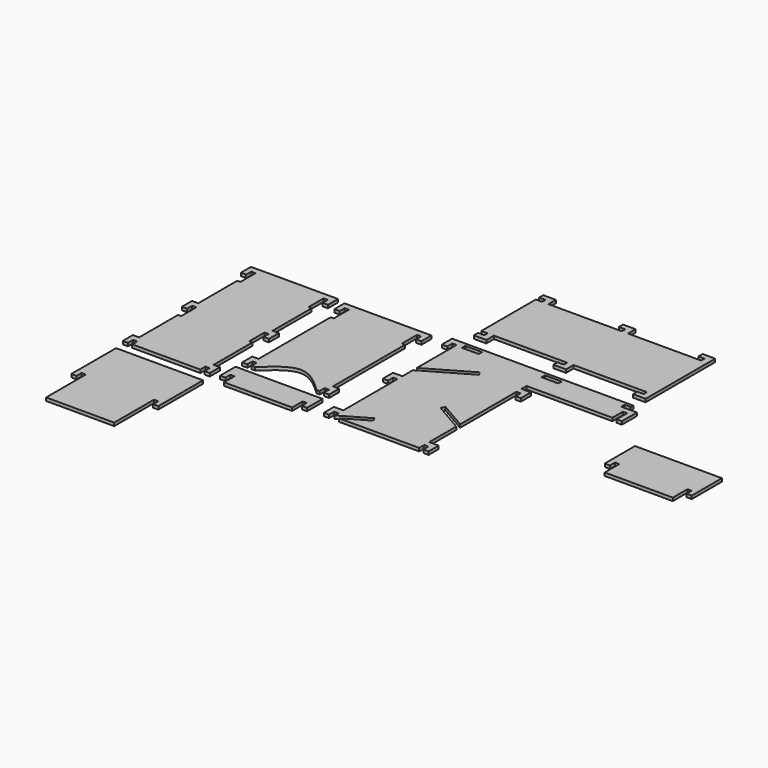
from build123d import *

# Parameters (mm, degrees)
F1_DEPTH = 3
F2_DEPTH = 3
F0_W     = 16
F0_H     = 4
F3_DEPTH = 3
F4_DEPTH = 3


with BuildPart() as f1:
    # F0 (on Top) → F1 (new body)
    with BuildSketch(Plane.XY):
        Polygon((-231.130471, -198.386263), (-231.130471, -245.736263), (-166.130471, -245.736263), (-166.130471, -198.386263), (-162.130471, -198.386263), (-162.130471, -204.386263), (-157.103619, -204.386263), (-157.103619, -151.036263), (-240.130471, -151.036263), (-240.130471, -204.386263), (-235.130471, -204.386263), (-235.130471, -198.386263), align=None)
    extrude(amount=F1_DEPTH)


with BuildPart() as f2:
    # F0 (on Top) → F2 (new body)
    with BuildSketch(Plane.XY):
        Polygon((-234.530405, -138.7419), (-169.530405, -138.7419), (-169.530405, -132.7419), (-165.530405, -132.7419), (-165.530405, -138.7419), (-160.530405, -138.7419), (-160.530405, -126.7419), (-166.530405, -126.7419), (-166.530405, -80.2419), (-169.530405, -80.2419), (-169.530405, -62.2419), (-165.530405, -62.2419), (-165.530405, -68.2419), (-160.503553, -68.2419), (-160.503553, -56.2419), (-166.530405, -56.2419), (-166.530405, -9.7419), (-169.530405, -9.7419), (-169.530405, 8.2581), (-165.530405, 8.2581), (-165.530405, 2.2581), (-160.503553, 2.2581), (-160.503553, 14.2581), (-243.530405, 14.2581), (-243.530405, 2.2581), (-238.530405, 2.2581), (-238.530405, 8.2581), (-234.530405, 8.2581), (-234.530405, -9.7419), (-237.530405, -9.7419), (-237.530405, -56.2419), (-243.530405, -56.2419), (-243.530405, -68.2419), (-238.530405, -68.2419), (-238.530405, -62.2419), (-234.530405, -62.2419), (-234.530405, -80.2419), (-237.530405, -80.2419), (-237.530405, -126.7419), (-243.530405, -126.7419), (-243.530405, -138.7419), (-238.530405, -138.7419), (-238.530405, -132.7419), (-234.530405, -132.7419), align=None)
    extrude(amount=F2_DEPTH)


with BuildPart() as f3:
    # F0 (on Top) → F3 (new body)
    with BuildSketch(Plane.XY):
        Polygon((118.848138, 17.368657), (-45.151862, 17.368657), (-54.151862, 17.368657), (-54.151862, 5.368657), (-49.151862, 5.368657), (-49.151862, 11.368657), (-45.151862, 11.368657), (-45.151862, -35.974066), (-3.989674, -12.209066), (-1.989674, -15.673167), (-45.151862, -40.592868), (-45.151862, -53.131343), (-54.151862, -53.131343), (-54.151862, -65.131343), (-49.151862, -65.131343), (-49.151862, -59.130682), (-45.151862, -59.130682), (-45.151862, -123.631343), (-54.151862, -123.631343), (-54.151862, -135.631343), (-49.151862, -135.631343), (-49.151862, -129.631343), (-45.151862, -129.631343), (-45.151862, -134.123611), (-19.171099, -119.123611), (-17.171099, -122.587713), (-39.76333, -135.631343), (36.848138, -135.631343), (36.848138, -129.631343), (40.848138, -129.631343), (40.848138, -135.631343), (45.848138, -135.631343), (45.848138, -123.631343), (36.848138, -123.631343), (36.848138, -91.399691), (8.867376, -75.244991), (10.867376, -71.780889), (36.848138, -86.780889), (36.848138, -19.631343), (40.848138, -19.631343), (40.848138, -25.719045), (45.848138, -25.631343), (45.848138, -13.631343), (36.848138, -13.631343), (36.848138, -7.631343), (118.848138, -7.631343), (118.848138, 4.868657), (122.848138, 4.868657), (122.848138, -7.631343), (127.848138, -7.631343), (127.848138, 10.368657), (112.848138, 10.368657), (112.848138, 14.368657), (118.709791, 14.368657), align=None)
        with Locations((-31.151862, 12.368657)):
            Rectangle(F0_W, F0_H, mode=Mode.SUBTRACT)
        Polygon((36.848138, 10.368657), (36.848138, 14.368657), (52.848138, 14.368657), (52.759487, 10.368657), align=None, mode=Mode.SUBTRACT)
    extrude(amount=F3_DEPTH)


with BuildPart() as f4:
    # F0 (on Top) → F4 (new body)
    with BuildSketch(Plane.XY):
        with BuildLine():
            Line((-143.392066, -104.227118), (-143.392066, -110.227118))
            Line((-143.392066, -110.227118), (-140.392066, -110.227118))
            add(Edge.make_bspline(
                [(-140.392066, -110.227118), (-131.894585, -102.449762), (-110.892066, -82.004474), (-89.889547, -102.449762), (-81.392066, -110.227118)],
                knots=[0, 0, 0, 0, 0.5, 1, 1, 1, 1], degree=3))
            Line((-81.392066, -110.227118), (-78.392066, -110.227118))
            Line((-78.392066, -110.227118), (-78.392066, -104.227118))
            Line((-78.392066, -104.227118), (-74.392066, -104.227118))
            Line((-74.392066, -104.227118), (-74.392066, -110.227118))
            Line((-74.392066, -110.227118), (-69.392066, -110.227118))
            Line((-69.392066, -110.227118), (-69.392066, -98.227118))
            Line((-69.392066, -98.227118), (-75.392066, -98.227118))
            Line((-75.392066, -98.227118), (-75.392066, -12.227118))
            Line((-75.392066, -12.227118), (-78.392066, -12.227118))
            Line((-78.392066, -12.227118), (-78.392066, 5.772882))
            Line((-78.392066, 5.772882), (-74.392066, 5.772882))
            Line((-74.392066, 5.772882), (-74.392066, -0.227118))
            Line((-74.392066, -0.227118), (-69.392066, -0.227118))
            Line((-69.392066, -0.227118), (-69.392066, 11.772882))
            Line((-69.392066, 11.772882), (-152.392066, 11.772882))
            Line((-152.392066, 11.772882), (-152.392066, -0.227118))
            Line((-152.392066, -0.227118), (-147.392066, -0.227118))
            Line((-147.392066, -0.227118), (-147.392066, 5.772882))
            Line((-147.392066, 5.772882), (-143.392066, 5.772882))
            Line((-143.392066, 5.772882), (-143.392066, -12.227118))
            Line((-143.392066, -12.227118), (-146.392066, -12.227118))
            Line((-146.392066, -12.227118), (-146.392066, -98.227118))
            Line((-146.392066, -98.227118), (-152.392066, -98.227118))
            Line((-152.392066, -98.227118), (-152.392066, -110.227118))
            Line((-152.392066, -110.227118), (-147.392066, -110.227118))
            Line((-147.392066, -110.227118), (-147.392066, -104.227118))
            Line((-147.392066, -104.227118), (-143.392066, -104.227118))
        make_face()
    extrude(amount=F4_DEPTH)


with BuildPart() as f4b:
    # F0 (on Top) → F4, piece 2 (new body)
    with BuildSketch(Plane.XY):
        Polygon((-44.905205, 105.659196), (-44.905205, 40.659196), (-38.905205, 40.659196), (-38.905205, 36.659196), (-44.905205, 36.659196), (-44.905205, 31.659196), (-32.905205, 31.659196), (-32.905205, 40.659196), (37.094795, 40.659196), (37.094795, 36.659196), (31.094795, 36.659196), (31.094795, 31.659196), (43.094795, 31.659196), (43.094795, 40.659196), (113.094795, 40.659196), (113.094795, 36.659196), (107.094795, 36.659196), (107.094795, 31.659196), (119.094795, 31.659196), (119.094795, 114.659196), (107.094795, 114.659196), (107.094795, 109.659196), (112.875297, 109.659196), (112.875297, 105.659196), (43.094795, 105.659196), (43.094795, 114.659196), (31.094795, 114.659196), (31.094795, 109.659196), (37.094795, 109.659196), (37.094795, 105.659196), (-32.905205, 105.659196), (-32.905205, 114.579205), (-44.905205, 114.579205), (-44.905205, 109.659196), (-38.905205, 109.659196), (-38.905205, 105.659196), align=None)
    extrude(amount=F4_DEPTH)


with BuildPart() as f4c:
    # F0 (on Top) → F4, piece 3 (new body)
    with BuildSketch(Plane.XY):
        Polygon((-68.830632, -118.789697), (-151.830632, -118.789697), (-151.830632, -137.289697), (-146.830632, -137.289697), (-146.830632, -131.289697), (-142.830632, -131.289697), (-142.830632, -143.789697), (-77.830632, -143.789697), (-77.830632, -131.289697), (-73.901128, -131.289697), (-73.901128, -137.289697), (-68.830632, -137.289697), align=None)
    extrude(amount=F4_DEPTH)


with BuildPart() as f4d:
    # F0 (on Top) → F4, piece 4 (new body)
    with BuildSketch(Plane.XY):
        Polygon((243.530405, -32.879844), (160.530405, -32.879844), (160.530405, -68.879844), (165.530405, -68.879844), (165.530405, -62.879844), (169.530405, -62.879844), (169.530405, -80.219844), (234.530405, -80.219844), (234.530405, -62.879844), (238.530405, -62.879844), (238.530405, -68.879844), (243.530405, -68.879844), align=None)
    extrude(amount=F4_DEPTH)


solid = Compound([f1.part, f2.part, f3.part, f4.part, f4b.part, f4c.part, f4d.part])
